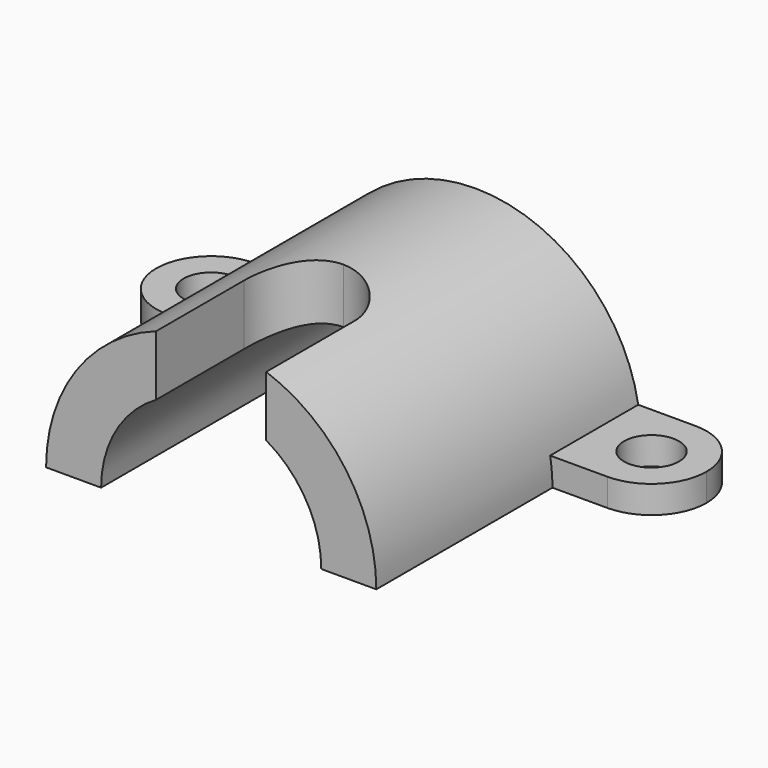
from build123d import *

# Parameters (mm, degrees)
F1_W      = 60
F1_H      = 60
F2_DEPTH  = 30
F4_DEPTH  = 60.001
F5_W      = 20
F5_H      = 20
F6_DEPTH  = 5
F7_W      = 20
F7_H      = 20
F8_DEPTH  = 5
F10_DEPTH = 20
F12_DEPTH = 40
F13_R     = 9.99999
F14_R     = 9.99999
F15_R     = 5
F16_DEPTH = 5.001
F17_R     = 5
F18_DEPTH = 5.001
F20_DEPTH = 30
F21_R     = 10
F22_R     = 9.99999


# Not quite as in the source:
# - a fillet or chamfer is up to 0.001 mm smaller than in the source, because OpenCascade refuses the exact size


with BuildPart() as f2:
    # F1 (on Top) → F2 (new body)
    with BuildSketch(Plane.XY):
        Rectangle(F1_W, F1_H)
    extrude(amount=F2_DEPTH)

    # F3 (on face) → F4 (cut, through all)
    with BuildSketch(Plane.XZ.offset(30)):
        with BuildLine():
            ThreePointArc((20, 0), (14.1421356237, 14.1421356237), (0, 20))
            Line((0, 20), (0, 0))
            Line((0, 0), (20, 0))
        make_face()
        with BuildLine():
            Line((0, 0), (0, 20))
            ThreePointArc((0, 20), (-14.1421356237, 14.1421356237), (-20, 0))
            Line((-20, 0), (0, 0))
        make_face()
    extrude(amount=-F4_DEPTH, mode=Mode.SUBTRACT)

    # F5 (on Top) → F6 (join)
    with BuildSketch(Plane.XY):
        with Locations((40, 20)):
            Rectangle(F5_W, F5_H)
    extrude(amount=F6_DEPTH)

    # F7 (on Top) → F8 (join)
    with BuildSketch(Plane.XY):
        with Locations((-40, 20)):
            Rectangle(F7_W, F7_H)
    extrude(amount=F8_DEPTH)

    # F9 (on face) → F10 (cut)
    with BuildSketch(Plane(origin=(0, 30, 0), x_dir=(-1, 0, 0), z_dir=(0, 1, 0))):
        with BuildLine():
            ThreePointArc((-29.5803989155, 5), (-19.3649167147, 22.9128784886), (4.28e-08, 30))
            Line((4.28e-08, 30), (-30, 30))
            Line((-30, 30), (-30, 5))
            Line((-30, 5), (-29.5803989155, 5))
        make_face()
        with BuildLine():
            ThreePointArc((4.28e-08, 30), (19.3649167474, 22.912878461), (29.5803989155, 5))
            Line((29.5803989155, 5), (30, 5))
            Line((30, 5), (30, 30))
            Line((30, 30), (4.28e-08, 30))
        make_face()
    extrude(amount=-F10_DEPTH, mode=Mode.SUBTRACT)

    # F11 (on face) → F12 (cut)
    with BuildSketch(Plane.XZ.offset(30)):
        with BuildLine():
            Line((-30, 30), (-30, 0))
            ThreePointArc((-30, 0), (-21.2132034683, 21.2132034029), (-9.24e-08, 30))
            Line((-9.24e-08, 30), (-30, 30))
        make_face()
        with BuildLine():
            ThreePointArc((-9.24e-08, 30), (21.2132034029, 21.2132034683), (30, 0))
            Line((30, 0), (30, 30))
            Line((30, 30), (-9.24e-08, 30))
        make_face()
    extrude(amount=-F12_DEPTH, mode=Mode.SUBTRACT)

    # F13 (radius 10 in the source; OpenCascade refuses exactly that, so slightly less here)
    f13_edges = [f2.edges().sort_by_distance(p)[0] for p in [
        (50, 30, 2.5),
        (50, 10, 2.5),
    ]]
    fillet(f13_edges, radius=F13_R)

    # F14 (radius 10 in the source; OpenCascade refuses exactly that, so slightly less here)
    f14_edges = [f2.edges().sort_by_distance(p)[0] for p in [
        (-50, 30, 2.5),
        (-50, 10, 2.5),
    ]]
    fillet(f14_edges, radius=F14_R)

    # F15 (on face) → F16 (cut, through all)
    with BuildSketch(Plane.XY.offset(5)):
        with Locations((-40, 20)):
            Circle(F15_R)
    extrude(amount=-F16_DEPTH, mode=Mode.SUBTRACT)

    # F17 (on face) → F18 (cut, through all)
    with BuildSketch(Plane.XY.offset(5)):
        with Locations((40, 20)):
            Circle(F17_R)
    extrude(amount=-F18_DEPTH, mode=Mode.SUBTRACT)

    # F19 (on face) → F20 (cut)
    with BuildSketch(Plane.XZ.offset(30)):
        with BuildLine():
            Line((10, 17.3205080757), (10, 28.2842712437))
            ThreePointArc((10.0000000012, 28.284271247), (1.3e-09, 30), (-9.9999999988, 28.2842712479))
            Line((-10, 28.2842712513), (-10, 17.3205080757))
            ThreePointArc((-10, 17.3205080757), (0, 20), (10, 17.3205080757))
        make_face()
    extrude(amount=-F20_DEPTH, mode=Mode.SUBTRACT)

    # F21
    f21_edges = [f2.edges().sort_by_distance(p)[0] for p in [
        (-10, 0, 22.80239),
    ]]
    fillet(f21_edges, radius=F21_R)

    # F22 (radius 10 in the source; OpenCascade refuses exactly that, so slightly less here)
    f22_edges = [f2.edges().sort_by_distance(p)[0] for p in [
        (10, 0, 22.80239),
    ]]
    fillet(f22_edges, radius=F22_R)


solid = f2.part
